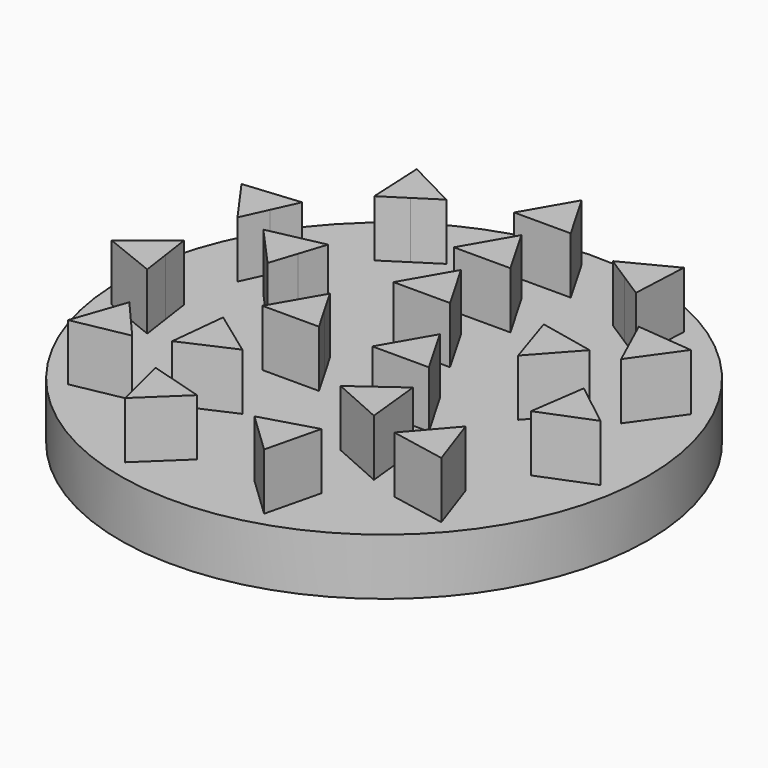
from build123d import *

# Parameters (mm, degrees)
F0_R     = 14
F1_DEPTH = 3
F3_DEPTH = 3


# Not quite as in the source:
# - a feature names something its author has since deleted; it is built from what else it names


with BuildPart() as f1:
    # F0 (on Top) → F1 (new body)
    with BuildSketch(Plane.XY):
        Circle(F0_R)
    extrude(amount=F1_DEPTH)

    # F2 (on face) → F3 (join)
    with BuildSketch(Plane.XY.offset(3)):
        Polygon((0, 6.5), (1.5, 6.5), (0, 9.0980762114), (-1.5, 6.5), align=None)
        Polygon((-6.6453928475, 0.582025689), (-6.1818673809, 2.0086103865), (-5.7183418644, 3.4351952379), (-8.6527846666, 2.8114601654), align=None)
        Polygon((-2.6070786483, -6.1402883419), (-3.8206041381, -5.2586104647), (-5.0341296315, -4.376932585), (-5.3477150213, -7.3604982711), align=None)
        Polygon((-6.9386088825, 8.0222008685), (-5.6767273349, 8.833162897), (-4.414848284, 9.6441233209), (-7.08135463, 11.0188028861), align=None)
        Polygon((0, 10.5), (1.5, 10.5), (0, 13.0980762114), (-1.5, 10.5), align=None)
        Polygon((4.3974313073, -9.6520773877), (2.9581918265, -10.0746762289), (1.5189523864, -10.4972750582), (3.6901545007, -12.5675120927), align=None)
        Polygon((-1.5189523864, -10.4972750582), (-2.9581918467, -10.074676223), (-4.3974313073, -9.6520773877), (-3.6901545007, -12.5675120927), align=None)
        Polygon((-6.9530794298, -8.009662068), (-7.9353704205, -6.8760378337), (-8.9176616316, -5.7424133449), (-9.8988655216, -8.577415801), align=None)
        Polygon((-10.1796528823, -2.9790379647), (-10.3931251437, -1.4943057747), (-10.6065973972, -0.009573639), (-12.9647566814, -1.8640505977), align=None)
        Polygon((0, 2.5), (1.5, 2.5), (0, 5.0980762114), (-1.5, 2.5), align=None)
        Polygon((-1.4150635095, -2.5490381057), (-2.1650632679, -1.2500004183), (-2.9150635095, 0.0490381057), (-4.4150635095, -2.5490381057), align=None)
        Polygon((2.9150635095, 0.0490381057), (2.1650632692, -1.2500004162), (1.4150635095, -2.5490381057), (4.4150635095, -2.5490381057), align=None)
        Polygon((8.9280134317, 5.7263056296), (9.5511359728, 4.3618575893), (10.1742584707, 2.9974096435), (11.9144291994, 5.4411374996), align=None)
        Polygon((5.7183418644, 3.4351952379), (6.1818673459, 2.0086104943), (6.6453928475, 0.582025689), (8.6527846666, 2.8114601654), align=None)
        Polygon((5.0341296315, -4.376932585), (3.8206041381, -5.2586104647), (2.6070786483, -6.1402883419), (5.3477150213, -7.3604982711), align=None)
        Polygon((8.9176616316, -5.7424133449), (7.9353705512, -6.8760376828), (6.9530794298, -8.009662068), (9.8988655216, -8.577415801), align=None)
        Polygon((10.6065973972, -0.009573639), (10.3931251437, -1.4943057747), (10.1796528823, -2.9790379647), (12.9647566814, -1.8640505977), align=None)
        Polygon((-10.1742584707, 2.9974096435), (-9.551135936, 4.3618576698), (-8.9280134317, 5.7263056296), (-11.9144291994, 5.4411374996), align=None)
        Polygon((4.414848284, 9.6441233209), (5.6767273496, 8.8331628876), (6.9386088825, 8.0222008685), (7.08135463, 11.0188028861), align=None)
    extrude(amount=F3_DEPTH)


solid = f1.part
